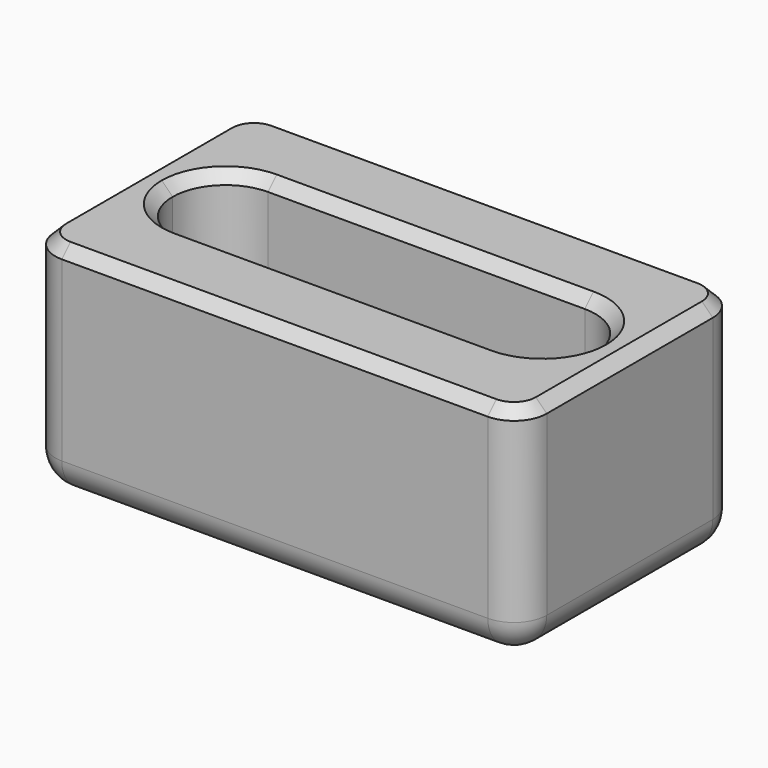
from build123d import *

# Parameters (mm, degrees)
F0_W         = 45
F0_H         = 25
F1_DEPTH     = 20.25
F3_DEPTH     = 10.8
F4_R         = 3
F5_SIZE      = 1
F6_TEXT_SIZE = 7.2518507327
F7_DEPTH     = 1


# Not quite as in the source:
# - Text() gives the source's letters only with a copy of the font that has no kerning and outlines rounded to 1/6400 em; it was checked with that copy


with BuildPart() as f1:
    # F0 (on Top) → F1 (new body)
    with BuildSketch(Plane.XY):
        Rectangle(F0_W, F0_H)
    extrude(amount=F1_DEPTH)

    # F2 (on face) → F3 (cut)
    with BuildSketch(Plane.XY.offset(20.25)):
        with BuildLine():
            Line((14.5, 4.85), (-14.5, 4.85))
            ThreePointArc((-14.5, 4.85), (-17.9294678888, 3.4294678888), (-19.35, 0))
            ThreePointArc((-19.35, 0), (-17.9294678888, -3.4294678888), (-14.5, -4.85))
            Line((-14.5, -4.85), (14.5, -4.85))
            ThreePointArc((14.5, -4.85), (17.9294678888, -3.4294678888), (19.35, 0))
            ThreePointArc((19.35, 0), (17.9294678888, 3.4294678888), (14.5, 4.85))
        make_face()
    extrude(amount=-F3_DEPTH, mode=Mode.SUBTRACT)

    # F4
    f4_edges = [f1.edges().sort_by_distance(p)[0] for p in [
        (-22.5, 0, 0),
        (0, -12.5, 0),
        (0, 12.5, 0),
        (22.5, 0, 0),
        (22.5, 12.5, 10.125),
        (22.5, -12.5, 10.125),
        (-22.5, -12.5, 10.125),
        (-22.5, 12.5, 10.125),
    ]]
    fillet(f4_edges, radius=F4_R)

    # F5
    f5_edges = [f1.edges().sort_by_distance(p)[0] for p in [
        (0, -12.5, 20.25),
        (19.35, 0, 20.25),
    ]]
    chamfer(f5_edges, length=F5_SIZE)

    # F6 (on face) → F7 (cut)
    with BuildSketch(Plane(origin=(0, 12.5, 0), x_dir=(-1, 0, 0), z_dir=(0, 1, 0))):
        with Locations((-14.7881719119, 7.162351251)):
            Text('EOS Tool', F6_TEXT_SIZE, font='Open Sans', text_align=(TextAlign.LEFT, TextAlign.BOTTOM))
    extrude(amount=-F7_DEPTH, mode=Mode.SUBTRACT)


solid = f1.part
